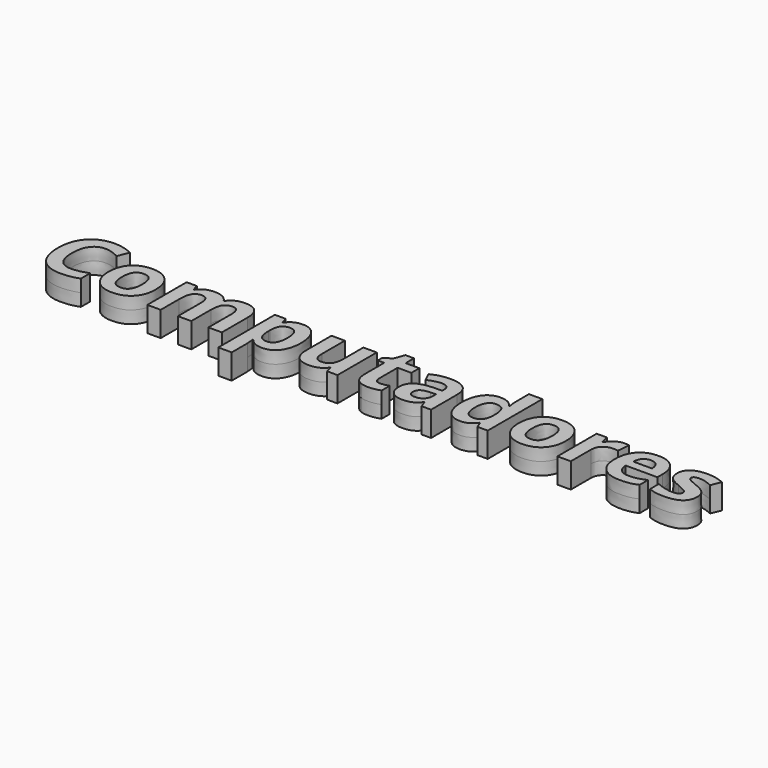
from build123d import *

# Parameters (mm, degrees)
F0_TEXT_SIZE = 72.049566855
F1_DEPTH     = 10


# Not quite as in the source:
# - Text() gives the source's letters only with a copy of the font that has no kerning and outlines rounded to 1/6400 em; it was checked with that copy


with BuildPart() as f1:
    # F0 (on Top) → F1 (new body, symmetric)
    with BuildSketch(Plane.XY):
        with Locations((-49.4721829891, -21.4312821627)):
            Text('Computadores', F0_TEXT_SIZE, font='Open Sans', font_style=FontStyle.BOLD, text_align=(TextAlign.LEFT, TextAlign.BOTTOM))
    extrude(amount=F1_DEPTH, both=True)


solid = f1.part
